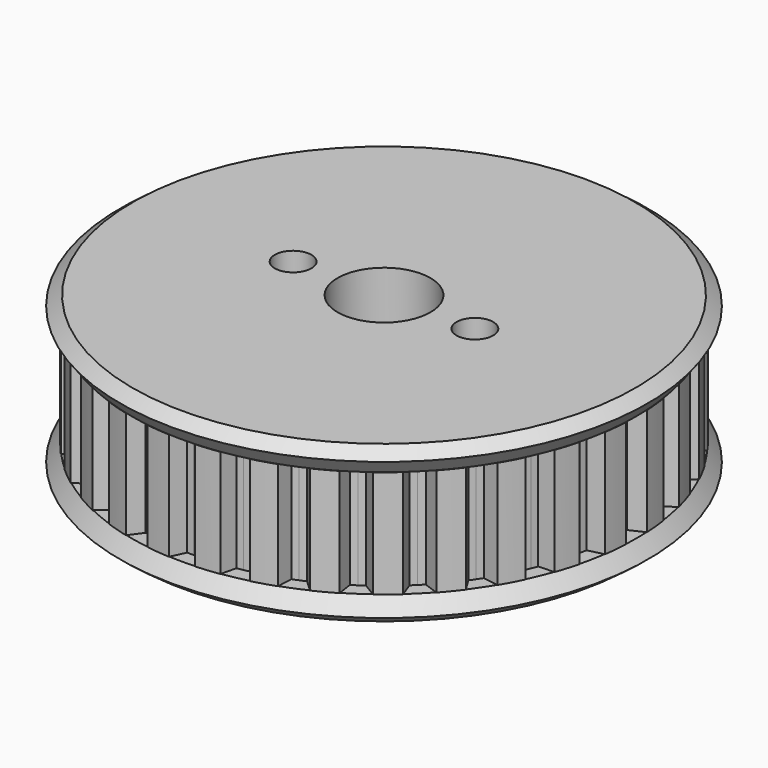
from build123d import *

# Parameters (mm, degrees)
F0_R            = 1.875
F0_R_2          = 4.75
F1_DEPTH        = 11
F2_DEPTH        = 11
F2_COPIES_COUNT = 32
F6_DEPTH        = 13.501
F6_DEPTH_BACK   = 2.501


# Not quite as in the source:
# - a pattern or mirror of a feature is missing from the dataset's text; its kind, count and spacing are read off the source's solid


with BuildPart() as f1:
    # F0 (on Top) → F1 (new body)
    with BuildSketch(Plane.XY):
        with BuildLine():
            Line((-0.65, 24.361330013), (-1.3373740713, 25.8354084658))
            ThreePointArc((-1.3373740713, 25.8354084658), (0, -25.87), (1.3373740713, 25.8354084658))
            Line((1.3373740713, 25.8354084658), (0.65, 24.361330013))
            ThreePointArc((0.65, 24.361330013), (0.3250289097, 24.3678324068), (0, 24.37))
            ThreePointArc((0, 24.37), (-0.3250289097, 24.3678324068), (-0.65, 24.361330013))
        make_face()
        with Locations((-9.3, 0)):
            Circle(F0_R, mode=Mode.SUBTRACT)
        Circle(F0_R_2, mode=Mode.SUBTRACT)
        with Locations((9.3, 0)):
            Circle(F0_R, mode=Mode.SUBTRACT)
        with BuildLine():
            ThreePointArc((1.3373740713, 25.8354084658), (0, 25.87), (-1.3373740713, 25.8354084658))
            Line((-1.3373740713, 25.8354084658), (-0.65, 24.361330013))
            ThreePointArc((-0.65, 24.361330013), (-0.3250289097, 24.3678324068), (0, 24.37))
            ThreePointArc((0, 24.37), (0.3250289097, 24.3678324068), (0.65, 24.361330013))
            Line((0.65, 24.361330013), (1.3373740713, 25.8354084658))
        make_face()
    extrude(amount=F1_DEPTH)

    # F0 (on Top) → F2 (cut, through all)
    with BuildSketch(Plane.XY):
        with BuildLine():
            ThreePointArc((1.3373740713, 25.8354084658), (0, 25.87), (-1.3373740713, 25.8354084658))
            Line((-1.3373740713, 25.8354084658), (-0.65, 24.361330013))
            ThreePointArc((-0.65, 24.361330013), (-0.3250289097, 24.3678324068), (0, 24.37))
            ThreePointArc((0, 24.37), (0.3250289097, 24.3678324068), (0.65, 24.361330013))
            Line((0.65, 24.361330013), (1.3373740713, 25.8354084658))
        make_face()
    f2 = extrude(amount=F2_DEPTH, mode=Mode.SUBTRACT)

    # F2_copies: F2 ×32 about axis
    f2_copies_axis = Axis((0, 0, 0), (0, 0, 1))
    for i in range(1, F2_COPIES_COUNT):
        add(f2.rotate(f2_copies_axis, i * 360 / F2_COPIES_COUNT), mode=Mode.SUBTRACT)

    # F4 (on Right) → F5 (revolve)
    with BuildSketch(Plane.YZ):
        Polygon((25.8354084658, 0), (0, 0), (0, -2.5), (25.7263896759, -2.5), (27, -1.5315389825), align=None)
        Polygon((25.8354084658, 11), (27, 12.5315389825), (25.7263896759, 13.5), (0, 13.5), (0, 11), align=None)
    revolve(axis=Axis((0, 0, -1.25), (0, 0, -1)))

    # F0 (on Top) → F6 (cut, two sides)
    with BuildSketch(Plane.XY) as f6_sk:
        with Locations((-9.3, 0)):
            Circle(F0_R)
        Circle(F0_R_2)
        with Locations((9.3, 0)):
            Circle(F0_R)
    extrude(amount=F6_DEPTH, mode=Mode.SUBTRACT)
    extrude(f6_sk.sketch, amount=-F6_DEPTH_BACK, mode=Mode.SUBTRACT)


solid = f1.part
